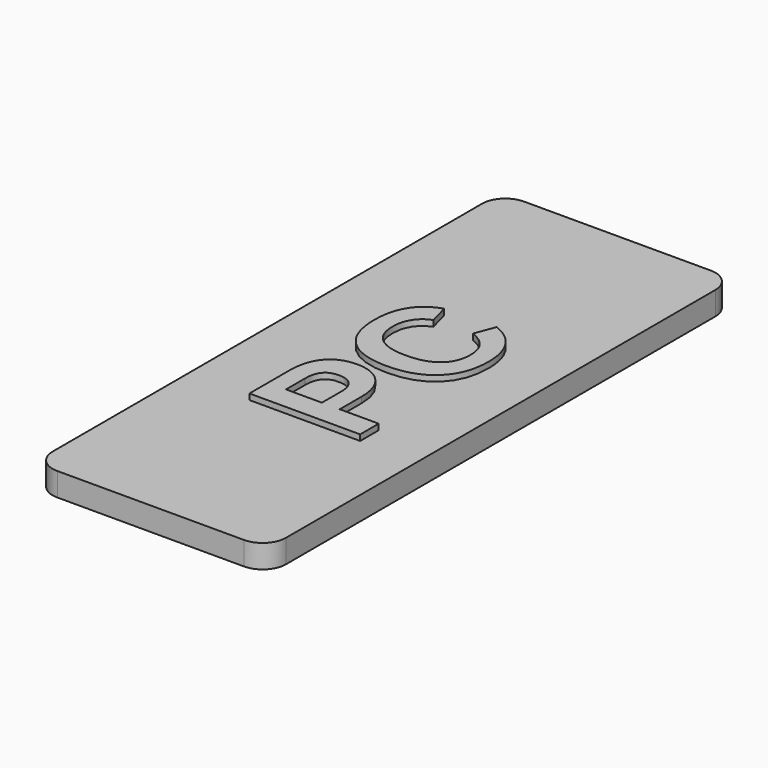
from build123d import *

# Parameters (mm, degrees)
F0_W         = 20
F0_H         = 50
F1_DEPTH     = 2
F2_R         = 2
F3_TEXT_SIZE = 13.7895914829
F4_DEPTH     = 2.5


# Not quite as in the source:
# - Text() gives the source's letters only with a copy of the font that has no kerning and outlines rounded to 1/6400 em; it was checked with that copy


with BuildPart() as f1:
    # F0 (on Top) → F1 (new body)
    with BuildSketch(Plane.XY):
        with Locations((-10, 0)):
            Rectangle(F0_W, F0_H)
    extrude(amount=F1_DEPTH)

    # F2
    f2_edges = [f1.edges().sort_by_distance(p)[0] for p in [
        (0, -25, 1),
        (-20, -25, 1),
        (0, 25, 1),
        (-20, 25, 1),
    ]]
    fillet(f2_edges, radius=F2_R)


with BuildPart() as f4:
    # F3 (on Top) → F4 (new body)
    with BuildSketch(Plane.XY):
        with Locations(Location((-4.8873303458, -9.868176405), (0, 0, 90))):
            Text('PC', F3_TEXT_SIZE, font='Arimo', font_style=FontStyle.BOLD, text_align=(TextAlign.LEFT, TextAlign.BOTTOM))
    extrude(amount=F4_DEPTH)


solid = Compound([f1.part, f4.part])
